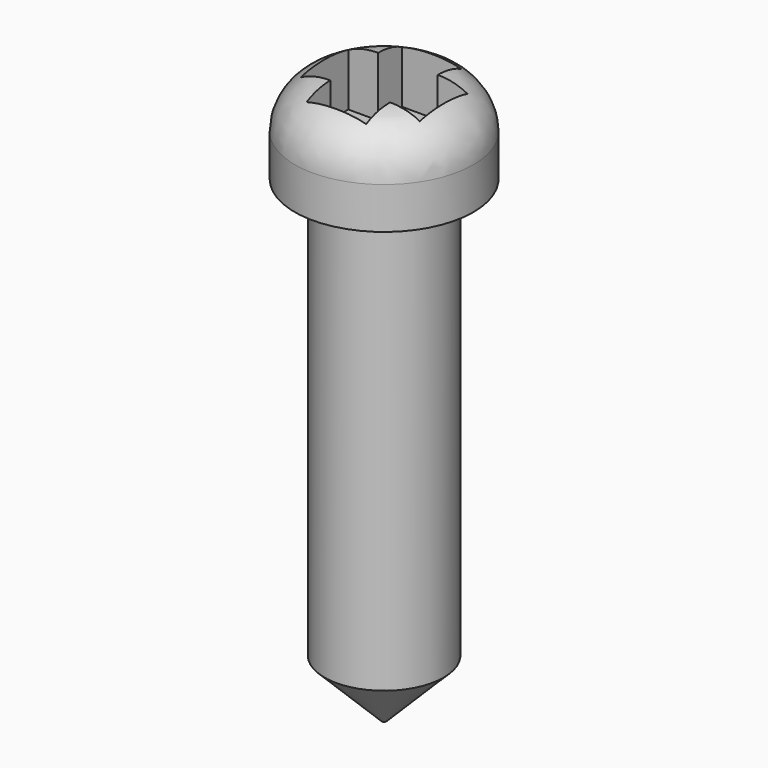
from build123d import *

# Parameters (mm, degrees)
F0_R     = 1.5875
F1_DEPTH = 12.7
F2_SIZE  = 1.524
F3_R     = 2.38125
F4_DEPTH = 2.38125
F5_W     = 1.5875
F5_H     = 0.79375
F5_W_2   = 0.79375
F5_H_2   = 1.5875
F6_DEPTH = 1.5875


# Not quite as in the source:
# - a fillet or chamfer that OpenCascade refuses, or shapes differently, is made with other operations: its cross-section is extruded or revolved along the edge and cut away or added


with BuildPart() as f1:
    # F0 (on Top) → F1 (new body)
    with BuildSketch(Plane.XY):
        Circle(F0_R)
    extrude(amount=F1_DEPTH)

    # F2
    f2_edges = [f1.edges().sort_by_distance(p)[0] for p in [
        (-1.5875, 0, 0),
    ]]
    chamfer(f2_edges, length=F2_SIZE)

    # F3 (on face) → F4 (join)
    with BuildSketch(Plane.XY.offset(12.7)):
        Circle(F3_R)
    extrude(amount=F4_DEPTH)

    # F5 (on face) → F6 (cut)
    with BuildSketch(Plane.XY.offset(15.08125)):
        with Locations((0, 1.190625)):
            Rectangle(F5_W, F5_H)
        with Locations((1.190625, 0)):
            Rectangle(F5_W_2, F5_H_2)
        Rectangle(F5_W, F5_H_2)
        with Locations((-1.190625, 0)):
            Rectangle(F5_W_2, F5_H_2)
        with Locations((0, -1.190625)):
            Rectangle(F5_W, F5_H)
    extrude(amount=-F6_DEPTH, mode=Mode.SUBTRACT)

    # F7: fillet of radius 1.27 on 1 edges, made by hand

    # F7_s1 → F7_t2 (revolve, cut)
    with BuildSketch(Plane.XZ):
        with BuildLine():
            ThreePointArc((2.38125, 13.81125), (2.0092756121, 14.7092756121), (1.11125, 15.08125))
            Line((1.11125, 15.08125), (2.38125, 15.08125))
            Line((2.38125, 15.08125), (2.38125, 13.81125))
        make_face()
    revolve(axis=Axis((0, 0, 15.08125), (0, 0, 1)), mode=Mode.SUBTRACT)


solid = f1.part
